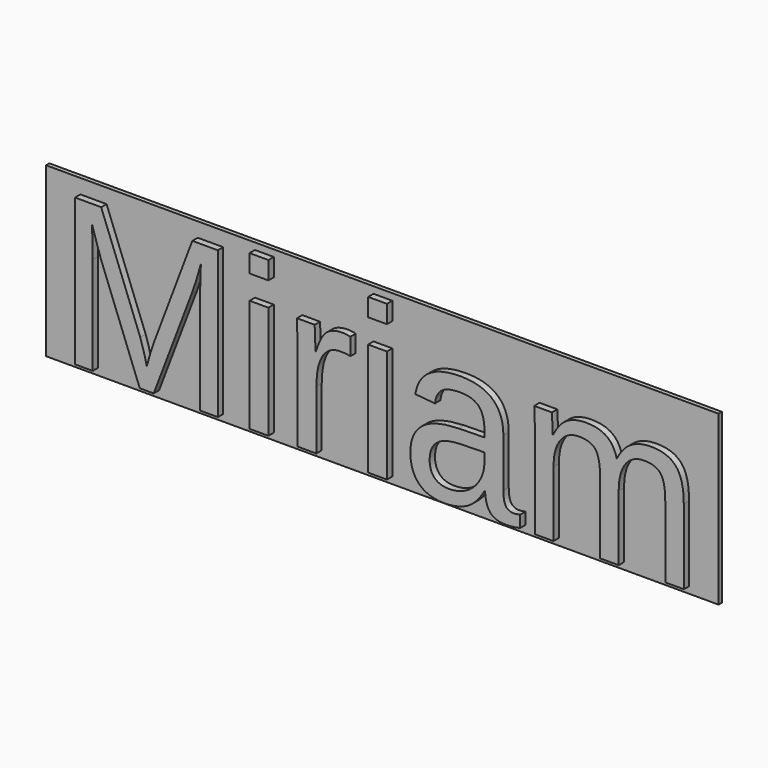
from build123d import *

# Parameters (mm, degrees)
F0_W         = 80
F0_H         = 20
F1_DEPTH     = 0.5
F2_TEXT_SIZE = 25.3992633791
F3_DEPTH     = 0.8


# Not quite as in the source:
# - Text() gives the source's letters only with a copy of the font that has no kerning and outlines rounded to 1/6400 em; it was checked with that copy


with BuildPart() as f1:
    # F0 (on Front) → F1 (new body)
    with BuildSketch(Plane.XZ):
        Rectangle(F0_W, F0_H)
    extrude(amount=-F1_DEPTH)

    # F2 (on face) → F3 (join)
    with BuildSketch(Plane.XZ):
        with Locations((-38.001999259, -9.1965887696)):
            Text('Miriam', F2_TEXT_SIZE, font='Arimo', text_align=(TextAlign.LEFT, TextAlign.BOTTOM))
    extrude(amount=F3_DEPTH)


solid = f1.part
